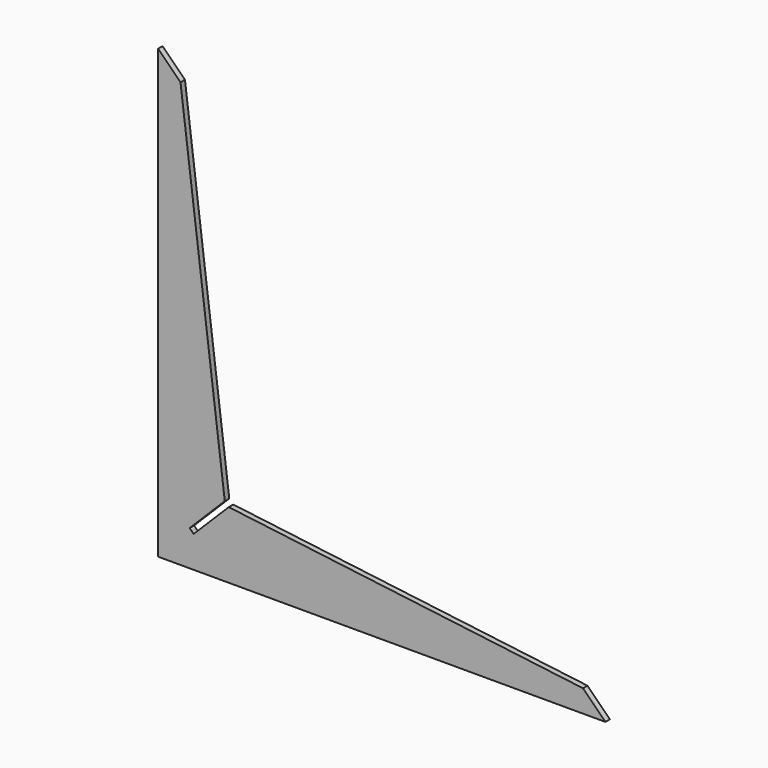
from build123d import *

# Parameters (mm, degrees)
F1_DEPTH = 12.7
F3_DEPTH = 25.4


# Not quite as in the source:
# - a length typed as a fraction of an inch, garbled in the dataset ("3 / 203.2 mm" for 3/8 in), is restored


with BuildPart() as f1:
    # F0 (on Front) → F1 (new body)
    with BuildSketch(Plane.XZ):
        Polygon((-313.2666666667, 601.1333333333), (-364.0666666667, 651.9333333333), (-364.0666666667, -364.0666666667), (651.9333333333, -364.0666666667), (601.1333333333, -313.2666666667), (-211.6666666667, -211.6666666667), align=None)
    extrude(amount=F1_DEPTH)

    # F2 (on face) → F3 (cut)
    with BuildSketch(Plane.XZ.offset(12.7)):
        Polygon((-292.3567947272, -283.3765386061), (-287.8666666667, -287.8666666667), (-283.3765386061, -292.3567947272), (-203.6842167813, -212.6644729023), (-212.6644729023, -203.6842167813), align=None)
    extrude(amount=-F3_DEPTH, mode=Mode.SUBTRACT)


solid = f1.part
